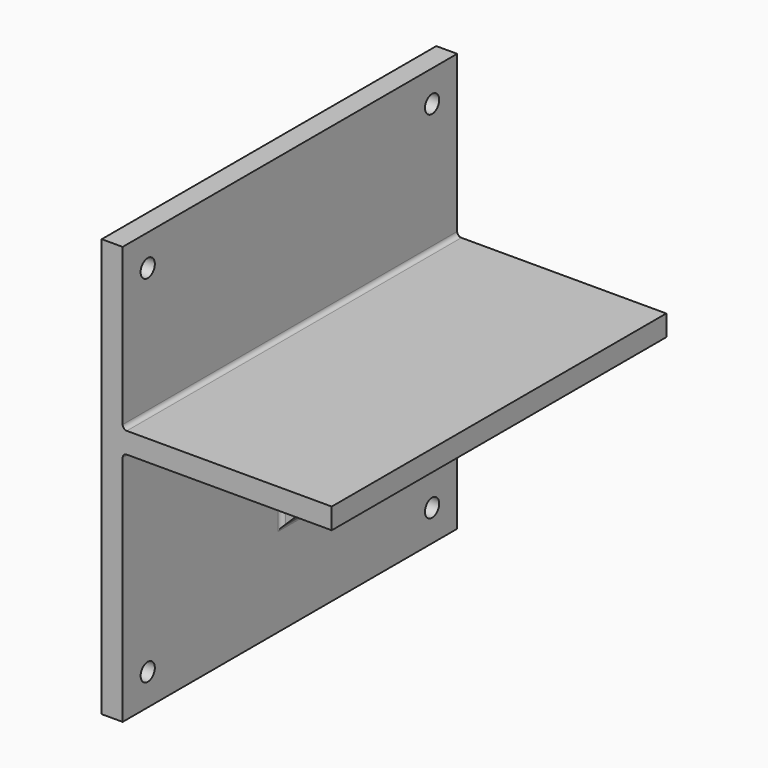
from build123d import *

# Parameters (mm, degrees)
F0_W         = 100
F0_H         = 10
F1_DEPTH     = 200
F2_W         = 10
F2_H         = 70
F3_DEPTH     = 70
F5_DEPTH     = 25
F6_R         = 4.25
F7_DEPTH     = 25
F8_DEPTH     = 25
F9_T1_DEPTH  = 200
F9_T3_DEPTH  = 93
F9_T5_DEPTH  = 93
F9_T7_DEPTH  = 10
F9_S11_W     = 2
F9_S11_H     = 2
F9_T12_DEPTH = 2
F9_S17_W     = 2
F9_S17_H     = 2
F9_T18_DEPTH = 2
F9_T24_DEPTH = 73
F9_T29_DEPTH = 73
F9_T34_DEPTH = 73
F9_T39_DEPTH = 73
F9_T45_DEPTH = 73
F9_T49_DEPTH = 12.0710678119
F9_T56_DEPTH = 12.0710678119
F9_T60_DEPTH = 73
F9_T67_DEPTH = 73
F9_T71_DEPTH = 12.0710678119
F9_T78_DEPTH = 12.0710678119
F9_T82_DEPTH = 73


# Not quite as in the source:
# - a fillet or chamfer that OpenCascade refuses, or shapes differently, is made with other operations: its cross-section is extruded or revolved along the edge and cut away or added


with BuildPart() as f1:
    # F0 (on Front) → F1 (new body)
    with BuildSketch(Plane.XZ):
        Polygon((-54.7254381291, 91.2093020976), (-64.7254381291, 91.2093020976), (-64.7254381291, -108.7906979024), (-54.7254381291, -108.7906979024), (-54.7254381291, 4.4093020976), (-54.7254381291, 14.4093020976), align=None)
        with Locations((-4.7254381291, 9.4093020976)):
            Rectangle(F0_W, F0_H)
    extrude(amount=F1_DEPTH)

    # F2 (on face) → F3 (join)
    with BuildSketch(Plane.YZ.offset(-54.7254381291)):
        with Locations((-100, -30.5906979024)):
            Rectangle(F2_W, F2_H)
    extrude(amount=F3_DEPTH)

    # F4 (on face) → F5 (cut)
    with BuildSketch(Plane.XZ.offset(105)):
        Polygon((15.2745618709, 4.4093020976), (-54.7254381291, -65.5906979024), (15.2745618709, -65.5906979024), align=None)
    extrude(amount=-F5_DEPTH, mode=Mode.SUBTRACT)

    # F6 (on face) → F7 (cut)
    with BuildSketch(Plane.YZ.offset(-54.7254381291)):
        with Locations((-15, 76.2093020976)):
            Circle(F6_R)
    extrude(amount=-F7_DEPTH, mode=Mode.SUBTRACT)

    # F6 (on face) → F8 (cut)
    with BuildSketch(Plane.YZ.offset(-54.7254381291)):
        with Locations((-185, 76.2093020976)):
            Circle(F6_R)
        with Locations((-15, 76.2093020976)):
            Circle(F6_R)
        with Locations((-185, -93.7906979024)):
            Circle(F6_R)
        with Locations((-15, -93.7906979024)):
            Circle(F6_R)
    extrude(amount=-F8_DEPTH, mode=Mode.SUBTRACT)

    # F9: fillet of radius 2 on 11 edges, made by hand

    # F9_s2 → F9_t1 (join)
    with BuildSketch(Plane.XZ):
        with BuildLine():
            ThreePointArc((-54.7254381291, 16.4093020976), (-54.1396516914, 14.9950885352), (-52.7254381291, 14.4093020976))
            Line((-52.7254381291, 14.4093020976), (-54.7254381291, 14.4093020976))
            Line((-54.7254381291, 14.4093020976), (-54.7254381291, 16.4093020976))
        make_face()
    extrude(amount=F9_T1_DEPTH)

    # F9_s4 → F9_t3 (join)
    with BuildSketch(Plane.XZ.offset(107)):
        with BuildLine():
            ThreePointArc((-54.7254381291, 2.4093020976), (-54.1396516914, 3.8235156599), (-52.7254381291, 4.4093020976))
            Line((-52.7254381291, 4.4093020976), (-54.7254381291, 4.4093020976))
            Line((-54.7254381291, 4.4093020976), (-54.7254381291, 2.4093020976))
        make_face()
    extrude(amount=F9_T3_DEPTH)

    # F9_s6 → F9_t5 (join)
    with BuildSketch(Plane.XZ):
        with BuildLine():
            ThreePointArc((-54.7254381291, 2.4093020976), (-54.1396516914, 3.8235156599), (-52.7254381291, 4.4093020976))
            Line((-52.7254381291, 4.4093020976), (-54.7254381291, 4.4093020976))
            Line((-54.7254381291, 4.4093020976), (-54.7254381291, 2.4093020976))
        make_face()
    extrude(amount=F9_T5_DEPTH)

    # F9_s8 → F9_t7 (join)
    with BuildSketch(Plane.XZ.offset(95)):
        with BuildLine():
            ThreePointArc((-54.7254381291, -66.4191250272), (-54.5731971941, -65.6537581625), (-54.1396516914, -65.0049114648))
            Line((-54.1396516914, -65.0049114648), (-54.7254381291, -65.5906979024))
            Line((-54.7254381291, -65.5906979024), (-54.7254381291, -66.4191250272))
        make_face()
        with BuildLine():
            ThreePointArc((16.1029889957, 4.4093020976), (15.3376221309, 4.2570611626), (14.6887754333, 3.8235156599))
            Line((14.6887754333, 3.8235156599), (15.2745618709, 4.4093020976))
            Line((15.2745618709, 4.4093020976), (16.1029889957, 4.4093020976))
        make_face()
    extrude(amount=F9_T7_DEPTH)


with BuildPart() as f9_tool10:
    # F9_s11 → F9_t12 (new body)
    with BuildSketch(Plane.XZ.offset(107)):
        with Locations((-53.7254381291, 3.4093020976)):
            Rectangle(F9_S11_W, F9_S11_H)
    extrude(amount=-F9_T12_DEPTH)

    # F9_s13 → F9_t14 (revolve, cut)
    with BuildSketch(Plane(origin=(-52.7254381291, -107, 2.4093020976), x_dir=(0.7071067812, 0, -0.7071067812), z_dir=(0.7071067812, 0, 0.7071067812))):
        with BuildLine():
            ThreePointArc((0, -2), (2, 0), (0, 2))
            Line((0, 2), (0, -2))
        make_face()
    revolve(axis=Axis((-52.7254381291, -107, 2.4093020976), (0, 1, 0)), mode=Mode.SUBTRACT)


with BuildPart() as f1_1:
    add(f1.part)

    # F9_t9: union F9_tool10
    add(f9_tool10.part)


with BuildPart() as f9_tool16:
    # F9_s17 → F9_t18 (new body)
    with BuildSketch(Plane.YZ.offset(-52.7254381291)):
        with Locations((-94, 3.4093020976)):
            Rectangle(F9_S17_W, F9_S17_H)
    extrude(amount=-F9_T18_DEPTH)

    # F9_s19 → F9_t20 (revolve, cut)
    with BuildSketch(Plane(origin=(-52.7254381291, -93, 2.4093020976), x_dir=(0, 0.7071067812, -0.7071067812), z_dir=(0, 0.7071067812, 0.7071067812))):
        with BuildLine():
            ThreePointArc((0, -2), (2, 0), (0, 2))
            Line((0, 2), (0, -2))
        make_face()
    revolve(axis=Axis((-52.7254381291, -93, 2.4093020976), (-1, 0, 0)), mode=Mode.SUBTRACT)


with BuildPart() as f1_2:
    add(f1_1.part)

    # F9_t15: union F9_tool16
    add(f9_tool16.part)


with BuildPart() as f9_tool22:
    # F9_s23 → F9_t24 (new body)
    with BuildSketch(Plane.XY.offset(-70.5906979024)):
        with BuildLine():
            ThreePointArc((-54.7254381291, -93), (-54.1396516914, -94.4142135624), (-52.7254381291, -95))
            Line((-52.7254381291, -95), (-54.7254381291, -95))
            Line((-54.7254381291, -95), (-54.7254381291, -93))
        make_face()
    extrude(amount=F9_T24_DEPTH)

    split(bisect_by=Plane(origin=(5.4326298867, 0, -5.4326298867), x_dir=(0, 1, 0), z_dir=(-0.7071067812, 0, 0.7071067812)), keep=Keep.TOP)


with BuildPart() as f1_3:
    add(f1_2.part)

    # F9_t21: union F9_tool22
    add(f9_tool22.part)


with BuildPart() as f9_tool27:
    # F9_s28 → F9_t29 (new body)
    with BuildSketch(Plane.XY.offset(2.4093020976)):
        with BuildLine():
            ThreePointArc((-54.7254381291, -107), (-54.1396516914, -105.5857864376), (-52.7254381291, -105))
            Line((-52.7254381291, -105), (-54.7254381291, -105))
            Line((-54.7254381291, -105), (-54.7254381291, -107))
        make_face()
    extrude(amount=-F9_T29_DEPTH)

    split(bisect_by=Plane(origin=(5.4326298867, 0, -5.4326298867), x_dir=(0, 1, 0), z_dir=(-0.7071067812, 0, 0.7071067812)), keep=Keep.TOP)


with BuildPart() as f1_4:
    add(f1_3.part)

    # F9_t26: union F9_tool27
    add(f9_tool27.part)


with BuildPart() as f9_tool32:
    # F9_s33 → F9_t34 (new body)
    with BuildSketch(Plane.YZ.offset(-52.7254381291)):
        with BuildLine():
            ThreePointArc((-93, 4.4093020976), (-94.4142135624, 3.8235156599), (-95, 2.4093020976))
            Line((-95, 2.4093020976), (-95, 4.4093020976))
            Line((-95, 4.4093020976), (-93, 4.4093020976))
        make_face()
    extrude(amount=F9_T34_DEPTH)

    split(bisect_by=Plane(origin=(5.4326298867, 0, -5.4326298867), x_dir=(0, 1, 0), z_dir=(-0.7071067812, 0, 0.7071067812)), keep=Keep.TOP)


with BuildPart() as f1_5:
    add(f1_4.part)

    # F9_t31: union F9_tool32
    add(f9_tool32.part)


with BuildPart() as f9_tool37:
    # F9_s38 → F9_t39 (new body)
    with BuildSketch(Plane.YZ.offset(-52.7254381291)):
        with BuildLine():
            ThreePointArc((-107, 4.4093020976), (-105.5857864376, 3.8235156599), (-105, 2.4093020976))
            Line((-105, 2.4093020976), (-105, 4.4093020976))
            Line((-105, 4.4093020976), (-107, 4.4093020976))
        make_face()
    extrude(amount=F9_T39_DEPTH)

    split(bisect_by=Plane(origin=(5.4326298867, 0, -5.4326298867), x_dir=(0, 1, 0), z_dir=(-0.7071067812, 0, 0.7071067812)), keep=Keep.TOP)


with BuildPart() as f1_6:
    add(f1_5.part)

    # F9_t36: union F9_tool37
    add(f9_tool37.part)


with BuildPart() as f9_tool43:
    # F9_s44 → F9_t45 (new body)
    with BuildSketch(Plane.XY.offset(-70.5906979024)):
        with BuildLine():
            ThreePointArc((-54.7254381291, -93), (-54.1396516914, -94.4142135624), (-52.7254381291, -95))
            Line((-52.7254381291, -95), (-54.7254381291, -95))
            Line((-54.7254381291, -95), (-54.7254381291, -93))
        make_face()
    extrude(amount=F9_T45_DEPTH)

    split(bisect_by=Plane(origin=(5.4326298867, 0, -5.4326298867), x_dir=(0, 1, 0), z_dir=(0.7071067812, 0, -0.7071067812)), keep=Keep.TOP)


with BuildPart() as f9_tool47:
    # F9_s48 → F9_t49 (new body)
    with BuildSketch(Plane.XZ.offset(105)):
        with BuildLine():
            ThreePointArc((-54.7254381291, -66.4191250272), (-54.5731971941, -65.6537581625), (-54.1396516914, -65.0049114648))
            Line((-54.1396516914, -65.0049114648), (-54.7254381291, -65.5906979024))
            Line((-54.7254381291, -65.5906979024), (-54.7254381291, -66.4191250272))
        make_face()
    extrude(amount=-F9_T49_DEPTH)

    split(bisect_by=Plane.XZ.offset(95), keep=Keep.BOTTOM)


with BuildPart() as f9_tool43_1:
    add(f9_tool43.part)

    # F9_t51: intersect F9_tool47
    add(f9_tool47.part, mode=Mode.INTERSECT)


with BuildPart() as f1_7:
    add(f1_6.part)

    # F9_t41: union F9_tool43
    add(f9_tool43_1.part)


with BuildPart() as f9_tool54:
    # F9_s55 → F9_t56 (new body)
    with BuildSketch(Plane.XZ.offset(107.0710678119)):
        with BuildLine():
            ThreePointArc((-54.7254381291, -66.4191250272), (-54.5731971941, -65.6537581625), (-54.1396516914, -65.0049114648))
            Line((-54.1396516914, -65.0049114648), (-54.7254381291, -65.5906979024))
            Line((-54.7254381291, -65.5906979024), (-54.7254381291, -66.4191250272))
        make_face()
    extrude(amount=-F9_T56_DEPTH)

    split(bisect_by=Plane.XZ.offset(105), keep=Keep.TOP)


with BuildPart() as f9_tool58:
    # F9_s59 → F9_t60 (new body)
    with BuildSketch(Plane.XY.offset(2.4093020976)):
        with BuildLine():
            ThreePointArc((-54.7254381291, -107), (-54.1396516914, -105.5857864376), (-52.7254381291, -105))
            Line((-52.7254381291, -105), (-54.7254381291, -105))
            Line((-54.7254381291, -105), (-54.7254381291, -107))
        make_face()
    extrude(amount=-F9_T60_DEPTH)

    split(bisect_by=Plane(origin=(5.4326298867, 0, -5.4326298867), x_dir=(0, 1, 0), z_dir=(0.7071067812, 0, -0.7071067812)), keep=Keep.TOP)


with BuildPart() as f9_tool54_1:
    add(f9_tool54.part)

    # F9_t62: intersect F9_tool58
    add(f9_tool58.part, mode=Mode.INTERSECT)


with BuildPart() as f1_8:
    add(f1_7.part)

    # F9_t52: union F9_tool54
    add(f9_tool54_1.part)


with BuildPart() as f9_tool65:
    # F9_s66 → F9_t67 (new body)
    with BuildSketch(Plane.YZ.offset(-52.7254381291)):
        with BuildLine():
            ThreePointArc((-93, 4.4093020976), (-94.4142135624, 3.8235156599), (-95, 2.4093020976))
            Line((-95, 2.4093020976), (-95, 4.4093020976))
            Line((-95, 4.4093020976), (-93, 4.4093020976))
        make_face()
    extrude(amount=F9_T67_DEPTH)

    split(bisect_by=Plane(origin=(5.4326298867, 0, -5.4326298867), x_dir=(0, 1, 0), z_dir=(0.7071067812, 0, -0.7071067812)), keep=Keep.TOP)


with BuildPart() as f9_tool69:
    # F9_s70 → F9_t71 (new body)
    with BuildSketch(Plane.XZ.offset(92.9289321881)):
        with BuildLine():
            ThreePointArc((16.1029889957, 4.4093020976), (15.3376221309, 4.2570611626), (14.6887754333, 3.8235156599))
            Line((14.6887754333, 3.8235156599), (15.2745618709, 4.4093020976))
            Line((15.2745618709, 4.4093020976), (16.1029889957, 4.4093020976))
        make_face()
    extrude(amount=F9_T71_DEPTH)

    split(bisect_by=Plane.XZ.offset(95), keep=Keep.BOTTOM)


with BuildPart() as f9_tool65_1:
    add(f9_tool65.part)

    # F9_t73: intersect F9_tool69
    add(f9_tool69.part, mode=Mode.INTERSECT)


with BuildPart() as f1_9:
    add(f1_8.part)

    # F9_t63: union F9_tool65
    add(f9_tool65_1.part)


with BuildPart() as f9_tool76:
    # F9_s77 → F9_t78 (new body)
    with BuildSketch(Plane.XZ.offset(95)):
        with BuildLine():
            ThreePointArc((16.1029889957, 4.4093020976), (15.3376221309, 4.2570611626), (14.6887754333, 3.8235156599))
            Line((14.6887754333, 3.8235156599), (15.2745618709, 4.4093020976))
            Line((15.2745618709, 4.4093020976), (16.1029889957, 4.4093020976))
        make_face()
    extrude(amount=F9_T78_DEPTH)

    split(bisect_by=Plane.XZ.offset(105), keep=Keep.TOP)


with BuildPart() as f9_tool80:
    # F9_s81 → F9_t82 (new body)
    with BuildSketch(Plane.YZ.offset(-52.7254381291)):
        with BuildLine():
            ThreePointArc((-107, 4.4093020976), (-105.5857864376, 3.8235156599), (-105, 2.4093020976))
            Line((-105, 2.4093020976), (-105, 4.4093020976))
            Line((-105, 4.4093020976), (-107, 4.4093020976))
        make_face()
    extrude(amount=F9_T82_DEPTH)

    split(bisect_by=Plane(origin=(5.4326298867, 0, -5.4326298867), x_dir=(0, 1, 0), z_dir=(0.7071067812, 0, -0.7071067812)), keep=Keep.TOP)


with BuildPart() as f9_tool76_1:
    add(f9_tool76.part)

    # F9_t84: intersect F9_tool80
    add(f9_tool80.part, mode=Mode.INTERSECT)


with BuildPart() as f1_10:
    add(f1_9.part)

    # F9_t74: union F9_tool76
    add(f9_tool76_1.part)


solid = f1_10.part
